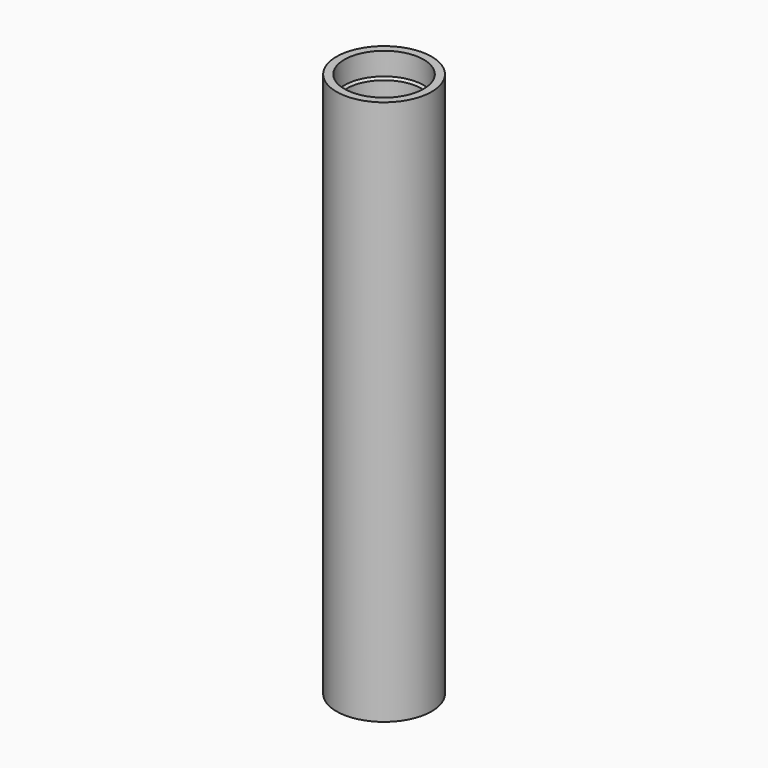
from build123d import *

# Parameters (mm, degrees)
F0_R         = 9.6
F0_R_2       = 8
F1_DEPTH     = 110
F0_R_3       = 7.55
F2_DEPTH     = 106
F3_DEPTH     = 4
F4_S5_R      = 8
F4_T6_DEPTH  = 14
F4_S11_R     = 8
F4_T12_DEPTH = 14


# Not quite as in the source:
# - a fillet or chamfer that OpenCascade refuses, or shapes differently, is made with other operations: its cross-section is extruded or revolved along the edge and cut away or added


with BuildPart() as f1:
    # F0 (on Top) → F1 (new body)
    with BuildSketch(Plane.XY):
        Circle(F0_R)
        Circle(F0_R_2, mode=Mode.SUBTRACT)
    extrude(amount=F1_DEPTH)

    # F0 (on Top) → F2 (join)
    with BuildSketch(Plane.XY):
        Circle(F0_R_2)
        Circle(F0_R_3, mode=Mode.SUBTRACT)
    extrude(amount=F2_DEPTH)

    # F0 (on Top) → F3 (cut)
    with BuildSketch(Plane.XY):
        Circle(F0_R_2)
        Circle(F0_R_3, mode=Mode.SUBTRACT)
    extrude(amount=F3_DEPTH, mode=Mode.SUBTRACT)

    # F4: chamfer of 1 on 2 edges, made by hand


with BuildPart() as f4_tool2:
    # F4_s3 → F4_t4 (revolve)
    with BuildSketch(Plane.XZ):
        Polygon((8.55, 4), (7.55, 5), (7.55, 4), align=None)
    revolve(axis=Axis((0, 0, 4), (0, 0, 1)))

    # F4_s5 → F4_t6 (intersect, symmetric)
    with BuildSketch(Plane.XY.offset(4.5)):
        Circle(F4_S5_R)
    extrude(amount=F4_T6_DEPTH, both=True, mode=Mode.INTERSECT)


with BuildPart() as f1_1:
    add(f1.part)

    # F4_t1: cut F4_tool2
    add(f4_tool2.part, mode=Mode.SUBTRACT)


with BuildPart() as f4_tool8:
    # F4_s9 → F4_t10 (revolve)
    with BuildSketch(Plane.XZ):
        Polygon((8.55, 106), (7.55, 105), (7.55, 106), align=None)
    revolve(axis=Axis((0, 0, 106), (0, 0, 1)))

    # F4_s11 → F4_t12 (intersect, symmetric)
    with BuildSketch(Plane.XY.offset(105.5)):
        Circle(F4_S11_R)
    extrude(amount=F4_T12_DEPTH, both=True, mode=Mode.INTERSECT)


with BuildPart() as f1_2:
    add(f1_1.part)

    # F4_t7: cut F4_tool8
    add(f4_tool8.part, mode=Mode.SUBTRACT)


solid = f1_2.part
